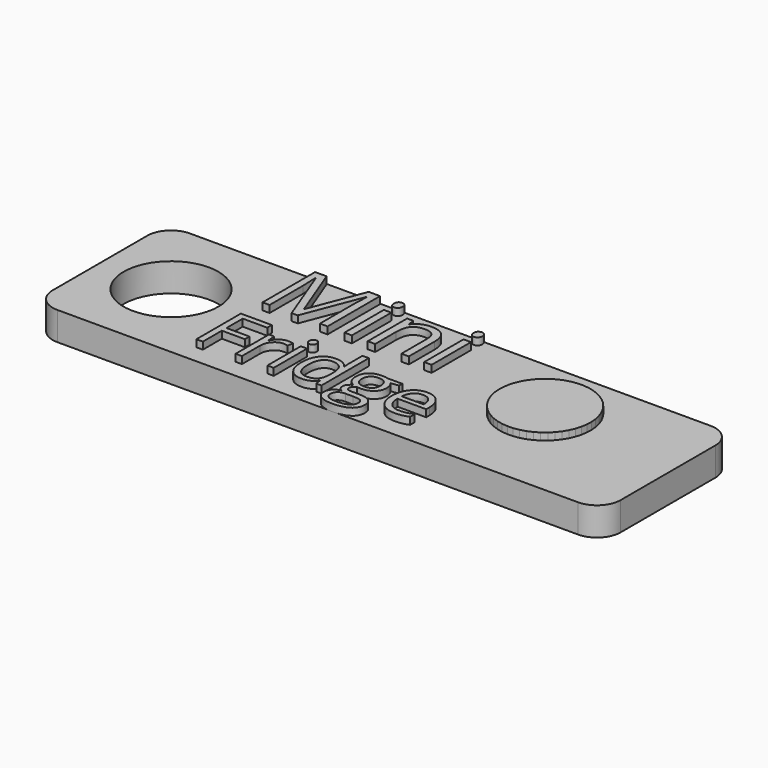
from build123d import *

# Parameters (mm, degrees)
F0_W           = 120
F0_H           = 35
F0_R           = 10
F1_DEPTH       = 6
F2_R           = 5
F3_TEXT_SIZE   = 19.4299910088
F3_TEXT_SIZE_2 = 16.455053507
F4_DEPTH       = 1.5


# Not quite as in the source:
# - Text() gives the source's letters only with a copy of the font that has no kerning and outlines rounded to 1/6400 em; it was checked with that copy


with BuildPart() as f1:
    # F0 (on Top) → F1 (new body)
    with BuildSketch(Plane.XY):
        Rectangle(F0_W, F0_H)
        with Locations((-45, 0)):
            Circle(F0_R, mode=Mode.SUBTRACT)
    extrude(amount=F1_DEPTH)

    # F2
    f2_edges = [f1.edges().sort_by_distance(p)[0] for p in [
        (60, -17.5, 3),
        (60, 17.5, 3),
        (-60, -17.5, 3),
        (-60, 17.5, 3),
    ]]
    fillet(f2_edges, radius=F2_R)

    # F3 (on face) → F4 (join)
    with BuildSketch(Plane.XY.offset(6)):
        Polygon((39.5426549973, -0.5529623489), (40.0217077671, 0.5529623489), (40.3583739442, 1.7102077329), (40.547344102, 2.9005233519), (40.5856380682, 4.1051372177), (40.472651924, 5.30505185), (40.2101675284, 6.4813438781), (39.8023244172, 7.6154624743), (39.2555545198, 8.6895219107), (38.5784807242, 9.6865836283), (37.7817808886, 10.5909233683), (36.8780194453, 11.3882791528), (35.8814492521, 12.0660762047), (34.8077868163, 12.6136252596), (33.673964436, 13.0222911419), (32.4978631673, 13.2856289463), (31.2980308298, 13.3994856786), (30.0933894963, 13.3620657499), (28.9029370802, 13.1739592949), (27.7454477272, 12.8381328647), (26.6391757358, 12.3598826429), (25.6015676763, 11.746750921), (24.6489872476, 11.0084071526), (23.7964572121, 10.15649546), (23.0574224777, 9.2044509995), (22.4435380636, 8.1672880809), (21.9644852938, 7.0613633831), (21.6278191166, 5.9041179991), (21.4388489588, 4.7138023801), (21.4005549927, 3.5091885143), (21.5135411369, 2.309273882), (21.7760255324, 1.1329818538), (22.1838686437, -0.0011367423), (22.730638541, -1.0751961787), (23.4077123366, -2.0722578963), (24.2044121723, -2.9765976363), (25.1081736156, -3.7739534208), (26.1047438088, -4.4517504727), (27.1784062445, -4.9992995276), (28.3122286249, -5.4079654099), (29.4883298936, -5.6713032144), (30.6881622311, -5.7851599466), (31.8928035646, -5.7477400179), (33.0832559807, -5.5596335629), (34.2407453337, -5.2238071327), (35.347017325, -4.7455569109), (36.3846253845, -4.132425189), (37.3372058133, -3.3940814206), (38.1897358488, -2.542169728), (38.9287705832, -1.5901252675), align=None)
        with Locations((-30.3739849478, 3.5104064737)):
            Text('Mini', F3_TEXT_SIZE, font='Open Sans', text_align=(TextAlign.LEFT, TextAlign.BOTTOM))
        with Locations((-30.3739849478, -13.6028439156)):
            Text('Fridge', F3_TEXT_SIZE_2, font='Open Sans', text_align=(TextAlign.LEFT, TextAlign.BOTTOM))
    extrude(amount=F4_DEPTH)


solid = f1.part
